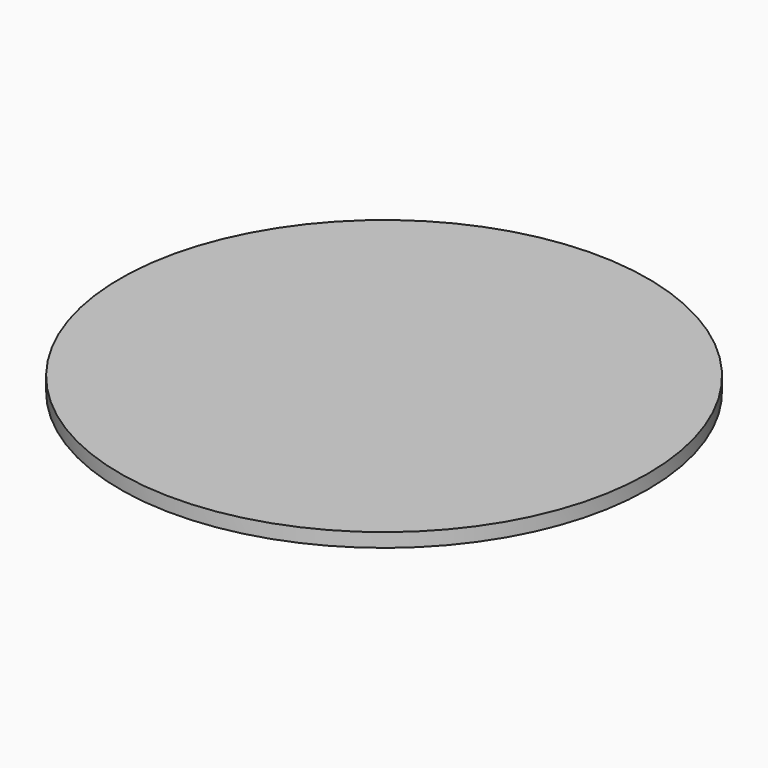
from build123d import *

# Parameters (mm, degrees)
F2_R     = 48.2408311773
F3_DEPTH = 2.54


# Not quite as in the source:
# - the program builds the solid bodies; features that only make, move or delete a surface that nothing else refers to are left out


with BuildPart() as f3:
    # F2 (on Top) → F3 (new body)
    with BuildSketch(Plane.XY):
        with Locations((-9.999348782, 16.2969231606)):
            Circle(F2_R)
    extrude(amount=F3_DEPTH)


solid = f3.part
